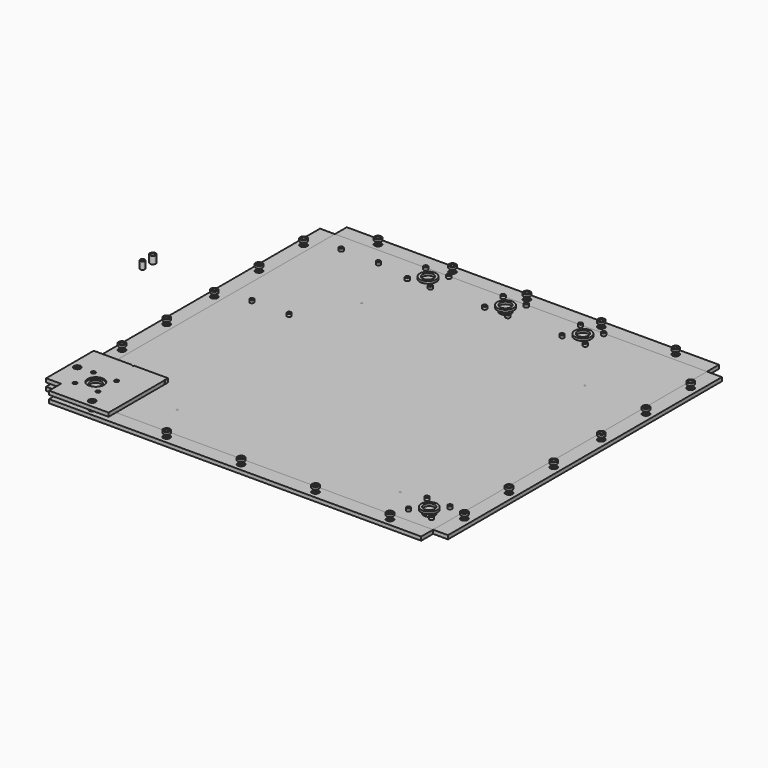
from build123d import *

# Parameters (mm, degrees)
F0_R      = 1.6
F0_R_2    = 2.6
F0_R_3    = 7.5
F0_R_4    = 1.25
F2_DEPTH  = 5
F3_R      = 2.75
F3_R_2    = 1.6
F3_R_3    = 4.6
F3_R_4    = 2.6
F4_DEPTH  = 1.5
F3_R_5    = 11
F3_R_6    = 7.5
F5_DEPTH  = 2
F6_R      = 3
F6_R_2    = 1.6
F7_DEPTH  = 5
F6_R_3    = 4
F6_R_4    = 2.6
F8_DEPTH  = 10
F10_W     = 500
F10_H     = 460
F10_R     = 7.5
F10_R_2   = 1.25
F10_W_2   = 65
F10_H_2   = 280
F11_DEPTH = 5
F12_DEPTH = 3
F14_R     = 4.6
F14_R_2   = 1.25
F14_R_3   = 2.75
F14_R_4   = 11
F15_DEPTH = 5


with BuildPart() as f2:
    # F0 (on Top) → F2 (new body)
    with BuildSketch(Plane.XY):
        Polygon((12.6355909109, 329.2870461196), (-237.3644090891, 329.2870461196), (-237.3644090891, 309.2870461196), (-257.3644090891, 309.2870461196), (-257.3644090891, -150.7129538804), (-237.3644090891, -150.7129538804), (-237.3644090891, -170.7129538804), (262.6355909109, -170.7129538804), (262.6355909109, -150.7129538804), (282.6355909109, -150.7129538804), (282.6355909109, 79.2870461196), (282.6355909109, 309.2870461196), (262.6355909109, 309.2870461196), (262.6355909109, 329.2870461196), align=None)
        with Locations((-226.8644090891, -140.2129538804)):
            Circle(F0_R, mode=Mode.SUBTRACT)
        with Locations((-195.8644090891, -140.2129538804)):
            Circle(F0_R, mode=Mode.SUBTRACT)
        with Locations((-247.3644090891, -110.7129538804)):
            Circle(F0_R_2, mode=Mode.SUBTRACT)
        with Locations((-226.8644090891, -109.2129538804)):
            Circle(F0_R, mode=Mode.SUBTRACT)
        with Locations((-211.3644090891, -124.7129538804)):
            Circle(F0_R_3, mode=Mode.SUBTRACT)
        with Locations((-195.8644090891, -109.2129538804)):
            Circle(F0_R, mode=Mode.SUBTRACT)
        with Locations((-187.3644090891, -160.7129538804)):
            Circle(F0_R_2, mode=Mode.SUBTRACT)
        with Locations((-204.3644090891, -70.8129538804)):
            Circle(F0_R_4, mode=Mode.SUBTRACT)
        with Locations((-156.6644090891, -77.1629538804)):
            Circle(F0_R_4, mode=Mode.SUBTRACT)
        with Locations((-87.3644090891, -160.7129538804)):
            Circle(F0_R_2, mode=Mode.SUBTRACT)
        with Locations((-247.3644090891, -35.7129538804)):
            Circle(F0_R_2, mode=Mode.SUBTRACT)
        with Locations((-204.3644090891, 4.1370461196)):
            Circle(F0_R_4, mode=Mode.SUBTRACT)
        with Locations((-156.6644090891, 5.3870461196)):
            Circle(F0_R_4, mode=Mode.SUBTRACT)
        with Locations((-247.3644090891, 39.2870461196)):
            Circle(F0_R_2, mode=Mode.SUBTRACT)
        with Locations((12.6355909109, -160.7129538804)):
            Circle(F0_R_2, mode=Mode.SUBTRACT)
        with Locations((112.6355909109, -160.7129538804)):
            Circle(F0_R_2, mode=Mode.SUBTRACT)
        with Locations((212.6355909109, -160.7129538804)):
            Circle(F0_R_2, mode=Mode.SUBTRACT)
        with Locations((221.1355909109, -140.2129538804)):
            Circle(F0_R, mode=Mode.SUBTRACT)
        with Locations((252.1355909109, -140.2129538804)):
            Circle(F0_R, mode=Mode.SUBTRACT)
        with Locations((236.6355909109, -124.7129538804)):
            Circle(F0_R_3, mode=Mode.SUBTRACT)
        with Locations((221.1355909109, -109.2129538804)):
            Circle(F0_R, mode=Mode.SUBTRACT)
        with Locations((252.1355909109, -109.2129538804)):
            Circle(F0_R, mode=Mode.SUBTRACT)
        with Locations((272.6355909109, -110.7129538804)):
            Circle(F0_R_2, mode=Mode.SUBTRACT)
        with Locations((272.6355909109, -35.7129538804)):
            Circle(F0_R_2, mode=Mode.SUBTRACT)
        with Locations((272.6355909109, 39.2870461196)):
            Circle(F0_R_2, mode=Mode.SUBTRACT)
        with Locations((-247.3644090891, 119.2870461196)):
            Circle(F0_R_2, mode=Mode.SUBTRACT)
        with Locations((-202.8644090891, 126.7870461196)):
            Circle(F0_R, mode=Mode.SUBTRACT)
        with Locations((-152.8644090891, 126.7870461196)):
            Circle(F0_R, mode=Mode.SUBTRACT)
        with Locations((-247.3644090891, 194.2870461196)):
            Circle(F0_R_2, mode=Mode.SUBTRACT)
        with Locations((-247.3644090891, 269.2870461196)):
            Circle(F0_R_2, mode=Mode.SUBTRACT)
        with Locations((-202.8644090891, 276.7870461196)):
            Circle(F0_R, mode=Mode.SUBTRACT)
        with Locations((-152.8644090891, 276.7870461196)):
            Circle(F0_R, mode=Mode.SUBTRACT)
        with Locations((-187.3644090891, 319.2870461196)):
            Circle(F0_R_2, mode=Mode.SUBTRACT)
        with Locations((-106.8644090891, 267.7870461196)):
            Circle(F0_R, mode=Mode.SUBTRACT)
        with Locations((-91.3644090891, 283.2870461196)):
            Circle(F0_R_3, mode=Mode.SUBTRACT)
        with Locations((-75.8644090891, 267.7870461196)):
            Circle(F0_R, mode=Mode.SUBTRACT)
        with Locations((-106.8644090891, 298.7870461196)):
            Circle(F0_R, mode=Mode.SUBTRACT)
        with Locations((-75.8644090891, 298.7870461196)):
            Circle(F0_R, mode=Mode.SUBTRACT)
        with Locations((-87.3644090891, 319.2870461196)):
            Circle(F0_R_2, mode=Mode.SUBTRACT)
        with Locations((-2.8644090891, 267.7870461196)):
            Circle(F0_R, mode=Mode.SUBTRACT)
        with Locations((-2.8644090891, 298.7870461196)):
            Circle(F0_R, mode=Mode.SUBTRACT)
        with Locations((272.6355909109, 119.2870461196)):
            Circle(F0_R_2, mode=Mode.SUBTRACT)
        with Locations((272.6355909109, 194.2870461196)):
            Circle(F0_R_2, mode=Mode.SUBTRACT)
        with Locations((28.1355909109, 267.7870461196)):
            Circle(F0_R, mode=Mode.SUBTRACT)
        with Locations((12.6355909109, 283.2870461196)):
            Circle(F0_R_3, mode=Mode.SUBTRACT)
        with Locations((28.1355909109, 298.7870461196)):
            Circle(F0_R, mode=Mode.SUBTRACT)
        with Locations((12.6355909109, 319.2870461196)):
            Circle(F0_R_2, mode=Mode.SUBTRACT)
        with Locations((101.1355909109, 267.7870461196)):
            Circle(F0_R, mode=Mode.SUBTRACT)
        with Locations((132.1355909109, 267.7870461196)):
            Circle(F0_R, mode=Mode.SUBTRACT)
        with Locations((116.6355909109, 283.2870461196)):
            Circle(F0_R_3, mode=Mode.SUBTRACT)
        with Locations((101.1355909109, 298.7870461196)):
            Circle(F0_R, mode=Mode.SUBTRACT)
        with Locations((112.6355909109, 319.2870461196)):
            Circle(F0_R_2, mode=Mode.SUBTRACT)
        with Locations((132.1355909109, 298.7870461196)):
            Circle(F0_R, mode=Mode.SUBTRACT)
        with Locations((212.6355909109, 319.2870461196)):
            Circle(F0_R_2, mode=Mode.SUBTRACT)
        with Locations((272.6355909109, 269.2870461196)):
            Circle(F0_R_2, mode=Mode.SUBTRACT)
    extrude(amount=F2_DEPTH)

    # F3 (on face) → F4 (cut)
    with BuildSketch(Plane.XY.offset(5)):
        with Locations((-202.8644090891, 276.7870461196)):
            Circle(F3_R)
        with Locations((-202.8644090891, 276.7870461196)):
            Circle(F3_R_2, mode=Mode.SUBTRACT)
        with Locations((-152.8644090891, 276.7870461196)):
            Circle(F3_R)
        with Locations((-152.8644090891, 276.7870461196)):
            Circle(F3_R_2, mode=Mode.SUBTRACT)
        with Locations((-106.8644090891, 267.7870461196)):
            Circle(F3_R)
        with Locations((-106.8644090891, 267.7870461196)):
            Circle(F3_R_2, mode=Mode.SUBTRACT)
        with Locations((272.6355909109, 269.2870461196)):
            Circle(F3_R_3)
        with Locations((272.6355909109, 269.2870461196)):
            Circle(F3_R_4, mode=Mode.SUBTRACT)
        with Locations((-106.8644090891, 298.7870461196)):
            Circle(F3_R)
        with Locations((-106.8644090891, 298.7870461196)):
            Circle(F3_R_2, mode=Mode.SUBTRACT)
        with Locations((-75.8644090891, 298.7870461196)):
            Circle(F3_R)
        with Locations((-75.8644090891, 298.7870461196)):
            Circle(F3_R_2, mode=Mode.SUBTRACT)
        with Locations((-75.8644090891, 267.7870461196)):
            Circle(F3_R)
        with Locations((-75.8644090891, 267.7870461196)):
            Circle(F3_R_2, mode=Mode.SUBTRACT)
        with Locations((101.1355909109, 298.7870461196)):
            Circle(F3_R)
        with Locations((101.1355909109, 298.7870461196)):
            Circle(F3_R_2, mode=Mode.SUBTRACT)
        with Locations((101.1355909109, 267.7870461196)):
            Circle(F3_R)
        with Locations((101.1355909109, 267.7870461196)):
            Circle(F3_R_2, mode=Mode.SUBTRACT)
        with Locations((132.1355909109, 298.7870461196)):
            Circle(F3_R)
        with Locations((132.1355909109, 298.7870461196)):
            Circle(F3_R_2, mode=Mode.SUBTRACT)
        with Locations((-202.8644090891, 126.7870461196)):
            Circle(F3_R)
        with Locations((-202.8644090891, 126.7870461196)):
            Circle(F3_R_2, mode=Mode.SUBTRACT)
        with Locations((-152.8644090891, 126.7870461196)):
            Circle(F3_R)
        with Locations((-152.8644090891, 126.7870461196)):
            Circle(F3_R_2, mode=Mode.SUBTRACT)
        with Locations((-187.3644090891, -160.7129538804)):
            Circle(F3_R_3)
        with Locations((-187.3644090891, -160.7129538804)):
            Circle(F3_R_4, mode=Mode.SUBTRACT)
        with Locations((-87.3644090891, -160.7129538804)):
            Circle(F3_R_3)
        with Locations((-87.3644090891, -160.7129538804)):
            Circle(F3_R_4, mode=Mode.SUBTRACT)
        with Locations((12.6355909109, -160.7129538804)):
            Circle(F3_R_3)
        with Locations((12.6355909109, -160.7129538804)):
            Circle(F3_R_4, mode=Mode.SUBTRACT)
        with Locations((112.6355909109, -160.7129538804)):
            Circle(F3_R_3)
        with Locations((112.6355909109, -160.7129538804)):
            Circle(F3_R_4, mode=Mode.SUBTRACT)
        with Locations((-195.8644090891, -109.2129538804)):
            Circle(F3_R)
        with Locations((-195.8644090891, -109.2129538804)):
            Circle(F3_R_2, mode=Mode.SUBTRACT)
        with Locations((-226.8644090891, -109.2129538804)):
            Circle(F3_R)
        with Locations((-226.8644090891, -109.2129538804)):
            Circle(F3_R_2, mode=Mode.SUBTRACT)
        with Locations((-226.8644090891, -140.2129538804)):
            Circle(F3_R)
        with Locations((-226.8644090891, -140.2129538804)):
            Circle(F3_R_2, mode=Mode.SUBTRACT)
        with Locations((-195.8644090891, -140.2129538804)):
            Circle(F3_R)
        with Locations((-195.8644090891, -140.2129538804)):
            Circle(F3_R_2, mode=Mode.SUBTRACT)
        with Locations((272.6355909109, 39.2870461196)):
            Circle(F3_R_3)
        with Locations((272.6355909109, 39.2870461196)):
            Circle(F3_R_4, mode=Mode.SUBTRACT)
        with Locations((272.6355909109, -35.7129538804)):
            Circle(F3_R_3)
        with Locations((272.6355909109, -35.7129538804)):
            Circle(F3_R_4, mode=Mode.SUBTRACT)
        with Locations((272.6355909109, -110.7129538804)):
            Circle(F3_R_3)
        with Locations((272.6355909109, -110.7129538804)):
            Circle(F3_R_4, mode=Mode.SUBTRACT)
        with Locations((221.1355909109, -109.2129538804)):
            Circle(F3_R)
        with Locations((221.1355909109, -109.2129538804)):
            Circle(F3_R_2, mode=Mode.SUBTRACT)
        with Locations((252.1355909109, -140.2129538804)):
            Circle(F3_R)
        with Locations((252.1355909109, -140.2129538804)):
            Circle(F3_R_2, mode=Mode.SUBTRACT)
        with Locations((221.1355909109, -140.2129538804)):
            Circle(F3_R)
        with Locations((221.1355909109, -140.2129538804)):
            Circle(F3_R_2, mode=Mode.SUBTRACT)
        with Locations((252.1355909109, -109.2129538804)):
            Circle(F3_R)
        with Locations((252.1355909109, -109.2129538804)):
            Circle(F3_R_2, mode=Mode.SUBTRACT)
        with Locations((272.6355909109, 119.2870461196)):
            Circle(F3_R_3)
        with Locations((272.6355909109, 119.2870461196)):
            Circle(F3_R_4, mode=Mode.SUBTRACT)
        with Locations((272.6355909109, 194.2870461196)):
            Circle(F3_R_3)
        with Locations((272.6355909109, 194.2870461196)):
            Circle(F3_R_4, mode=Mode.SUBTRACT)
        with Locations((132.1355909109, 267.7870461196)):
            Circle(F3_R)
        with Locations((132.1355909109, 267.7870461196)):
            Circle(F3_R_2, mode=Mode.SUBTRACT)
        with Locations((212.6355909109, -160.7129538804)):
            Circle(F3_R_3)
        with Locations((212.6355909109, -160.7129538804)):
            Circle(F3_R_4, mode=Mode.SUBTRACT)
        with Locations((-2.8644090891, 298.7870461196)):
            Circle(F3_R)
        with Locations((-2.8644090891, 298.7870461196)):
            Circle(F3_R_2, mode=Mode.SUBTRACT)
        with Locations((28.1355909109, 298.7870461196)):
            Circle(F3_R)
        with Locations((28.1355909109, 298.7870461196)):
            Circle(F3_R_2, mode=Mode.SUBTRACT)
        with Locations((28.1355909109, 267.7870461196)):
            Circle(F3_R)
        with Locations((28.1355909109, 267.7870461196)):
            Circle(F3_R_2, mode=Mode.SUBTRACT)
        with Locations((-2.8644090891, 267.7870461196)):
            Circle(F3_R)
        with Locations((-2.8644090891, 267.7870461196)):
            Circle(F3_R_2, mode=Mode.SUBTRACT)
    extrude(amount=-F4_DEPTH, mode=Mode.SUBTRACT)

    # F3 (on face) → F5 (cut)
    with BuildSketch(Plane.XY.offset(5)):
        with Locations((-211.3644090891, -124.7129538804)):
            Circle(F3_R_5)
        with Locations((-211.3644090891, -124.7129538804)):
            Circle(F3_R_6, mode=Mode.SUBTRACT)
        with Locations((236.6355909109, -124.7129538804)):
            Circle(F3_R_5)
        with Locations((236.6355909109, -124.7129538804)):
            Circle(F3_R_6, mode=Mode.SUBTRACT)
        with Locations((116.6355909109, 283.2870461196)):
            Circle(F3_R_5)
        with Locations((116.6355909109, 283.2870461196)):
            Circle(F3_R_6, mode=Mode.SUBTRACT)
        with Locations((-91.3644090891, 283.2870461196)):
            Circle(F3_R_5)
        with Locations((-91.3644090891, 283.2870461196)):
            Circle(F3_R_6, mode=Mode.SUBTRACT)
        with Locations((12.6355909109, 283.2870461196)):
            Circle(F3_R_5)
        with Locations((12.6355909109, 283.2870461196)):
            Circle(F3_R_6, mode=Mode.SUBTRACT)
        with Locations((-247.3644090891, 269.2870461196)):
            Circle(F3_R_3)
        with Locations((-247.3644090891, 269.2870461196)):
            Circle(F3_R_4, mode=Mode.SUBTRACT)
        with Locations((-187.3644090891, 319.2870461196)):
            Circle(F3_R_3)
        with Locations((-187.3644090891, 319.2870461196)):
            Circle(F3_R_4, mode=Mode.SUBTRACT)
        with Locations((-87.3644090891, 319.2870461196)):
            Circle(F3_R_3)
        with Locations((-87.3644090891, 319.2870461196)):
            Circle(F3_R_4, mode=Mode.SUBTRACT)
        with Locations((12.6355909109, 319.2870461196)):
            Circle(F3_R_3)
        with Locations((12.6355909109, 319.2870461196)):
            Circle(F3_R_4, mode=Mode.SUBTRACT)
        with Locations((112.6355909109, 319.2870461196)):
            Circle(F3_R_3)
        with Locations((112.6355909109, 319.2870461196)):
            Circle(F3_R_4, mode=Mode.SUBTRACT)
        with Locations((212.6355909109, 319.2870461196)):
            Circle(F3_R_3)
        with Locations((212.6355909109, 319.2870461196)):
            Circle(F3_R_4, mode=Mode.SUBTRACT)
        with Locations((272.6355909109, 269.2870461196)):
            Circle(F3_R_3)
        with Locations((272.6355909109, 269.2870461196)):
            Circle(F3_R_4, mode=Mode.SUBTRACT)
        with Locations((-247.3644090891, 194.2870461196)):
            Circle(F3_R_3)
        with Locations((-247.3644090891, 194.2870461196)):
            Circle(F3_R_4, mode=Mode.SUBTRACT)
        with Locations((-247.3644090891, 119.2870461196)):
            Circle(F3_R_3)
        with Locations((-247.3644090891, 119.2870461196)):
            Circle(F3_R_4, mode=Mode.SUBTRACT)
        with Locations((-247.3644090891, 39.2870461196)):
            Circle(F3_R_3)
        with Locations((-247.3644090891, 39.2870461196)):
            Circle(F3_R_4, mode=Mode.SUBTRACT)
        with Locations((-247.3644090891, -35.7129538804)):
            Circle(F3_R_3)
        with Locations((-247.3644090891, -35.7129538804)):
            Circle(F3_R_4, mode=Mode.SUBTRACT)
        with Locations((-247.3644090891, -110.7129538804)):
            Circle(F3_R_3)
        with Locations((-247.3644090891, -110.7129538804)):
            Circle(F3_R_4, mode=Mode.SUBTRACT)
        with Locations((-187.3644090891, -160.7129538804)):
            Circle(F3_R_3)
        with Locations((-187.3644090891, -160.7129538804)):
            Circle(F3_R_4, mode=Mode.SUBTRACT)
        with Locations((-87.3644090891, -160.7129538804)):
            Circle(F3_R_3)
        with Locations((-87.3644090891, -160.7129538804)):
            Circle(F3_R_4, mode=Mode.SUBTRACT)
        with Locations((12.6355909109, -160.7129538804)):
            Circle(F3_R_3)
        with Locations((12.6355909109, -160.7129538804)):
            Circle(F3_R_4, mode=Mode.SUBTRACT)
        with Locations((112.6355909109, -160.7129538804)):
            Circle(F3_R_3)
        with Locations((112.6355909109, -160.7129538804)):
            Circle(F3_R_4, mode=Mode.SUBTRACT)
        with Locations((272.6355909109, 39.2870461196)):
            Circle(F3_R_3)
        with Locations((272.6355909109, 39.2870461196)):
            Circle(F3_R_4, mode=Mode.SUBTRACT)
        with Locations((272.6355909109, -35.7129538804)):
            Circle(F3_R_3)
        with Locations((272.6355909109, -35.7129538804)):
            Circle(F3_R_4, mode=Mode.SUBTRACT)
        with Locations((272.6355909109, -110.7129538804)):
            Circle(F3_R_3)
        with Locations((272.6355909109, -110.7129538804)):
            Circle(F3_R_4, mode=Mode.SUBTRACT)
        with Locations((272.6355909109, 119.2870461196)):
            Circle(F3_R_3)
        with Locations((272.6355909109, 119.2870461196)):
            Circle(F3_R_4, mode=Mode.SUBTRACT)
        with Locations((272.6355909109, 194.2870461196)):
            Circle(F3_R_3)
        with Locations((272.6355909109, 194.2870461196)):
            Circle(F3_R_4, mode=Mode.SUBTRACT)
        with Locations((212.6355909109, -160.7129538804)):
            Circle(F3_R_3)
        with Locations((212.6355909109, -160.7129538804)):
            Circle(F3_R_4, mode=Mode.SUBTRACT)
        with Locations((272.6355909109, -110.7129538804)):
            Circle(F3_R_4)
        with Locations((212.6355909109, -160.7129538804)):
            Circle(F3_R_4)
        with Locations((272.6355909109, -35.7129538804)):
            Circle(F3_R_4)
        with Locations((112.6355909109, -160.7129538804)):
            Circle(F3_R_4)
        with Locations((272.6355909109, 39.2870461196)):
            Circle(F3_R_4)
        with Locations((272.6355909109, 119.2870461196)):
            Circle(F3_R_4)
        with Locations((272.6355909109, 194.2870461196)):
            Circle(F3_R_4)
        with Locations((272.6355909109, 269.2870461196)):
            Circle(F3_R_4)
        with Locations((-187.3644090891, -160.7129538804)):
            Circle(F3_R_4)
        with Locations((-87.3644090891, -160.7129538804)):
            Circle(F3_R_4)
        with Locations((12.6355909109, -160.7129538804)):
            Circle(F3_R_4)
    extrude(amount=-F5_DEPTH, mode=Mode.SUBTRACT)


with BuildPart() as f7:
    # F6 (on Top) → F7 (new body)
    with BuildSketch(Plane.XY):
        with Locations((-351.8798351288, 129.4269926766)):
            Circle(F6_R)
        with Locations((-351.8798351288, 129.4269926766)):
            Circle(F6_R_2, mode=Mode.SUBTRACT)
    extrude(amount=F7_DEPTH)


with BuildPart() as f7b:
    # F6 (on Top) → F7, piece 2 (new body)
    with BuildSketch(Plane.XY):
        with Locations((-351.8798351288, 146.7694063903)):
            Circle(F6_R_3)
        with Locations((-351.8798351288, 146.7694063903)):
            Circle(F6_R_4, mode=Mode.SUBTRACT)
    extrude(amount=F7_DEPTH)


with BuildPart() as f8:
    # F6 (on Top) → F8 (new body)
    with BuildSketch(Plane.XY):
        with Locations((-351.8798351288, 146.7694063903)):
            Circle(F6_R_3)
        with Locations((-351.8798351288, 146.7694063903)):
            Circle(F6_R_4, mode=Mode.SUBTRACT)
    extrude(amount=F8_DEPTH)


with BuildPart() as f8b:
    # F6 (on Top) → F8, piece 2 (new body)
    with BuildSketch(Plane.XY):
        with Locations((-351.8798351288, 129.4269926766)):
            Circle(F6_R)
        with Locations((-351.8798351288, 129.4269926766)):
            Circle(F6_R_2, mode=Mode.SUBTRACT)
    extrude(amount=F8_DEPTH)


with BuildPart() as f11:
    # F10 (on face) → F11 (new body)
    with BuildSketch(Plane.XY):
        with Locations((12.6355909109, 79.2870461196)):
            Rectangle(F10_W, F10_H)
        with Locations((-211.3644090891, -124.7129538804)):
            Circle(F10_R, mode=Mode.SUBTRACT)
        with Locations((236.6355909109, -124.7129538804)):
            Circle(F10_R, mode=Mode.SUBTRACT)
        Polygon((-128.5639107227, -110.7129538804), (-127.3644090891, 209.2870461196), (192.6355909109, 209.2870461196), (192.6355909109, -110.7129538804), (-117.3644090891, -110.7129538804), align=None, mode=Mode.SUBTRACT)
        with Locations((12.6355909109, 283.2870461196)):
            Circle(F10_R, mode=Mode.SUBTRACT)
        Polygon((192.6355909109, 209.2870461196), (-127.3644090891, 209.2870461196), (-128.5639107227, -110.7129538804), (-117.3644090891, -110.7129538804), (192.6355909109, -110.7129538804), align=None)
        with Locations((-117.3644090891, -105.7129538804)):
            Circle(F10_R_2, mode=Mode.SUBTRACT)
        with Locations((-74.8644090891, 49.2870461196)):
            Rectangle(F10_W_2, F10_H_2, mode=Mode.SUBTRACT)
        with Locations((182.6355909109, -105.7129538804)):
            Circle(F10_R_2, mode=Mode.SUBTRACT)
        with Locations((-117.3644090891, 204.2870461196)):
            Circle(F10_R_2, mode=Mode.SUBTRACT)
        with Locations((182.6355909109, 204.2870461196)):
            Circle(F10_R_2, mode=Mode.SUBTRACT)
        with Locations((-74.8644090891, 49.2870461196)):
            Rectangle(F10_W_2, F10_H_2)
    extrude(amount=F11_DEPTH)


with BuildPart() as f12:
    # F10 (on face) → F12 (new body)
    with BuildSketch(Plane.XY):
        Polygon((192.6355909109, 209.2870461196), (-127.3644090891, 209.2870461196), (-128.5639107227, -110.7129538804), (-117.3644090891, -110.7129538804), (192.6355909109, -110.7129538804), align=None)
        with Locations((-117.3644090891, -105.7129538804)):
            Circle(F10_R_2, mode=Mode.SUBTRACT)
        with Locations((-74.8644090891, 49.2870461196)):
            Rectangle(F10_W_2, F10_H_2, mode=Mode.SUBTRACT)
        with Locations((182.6355909109, -105.7129538804)):
            Circle(F10_R_2, mode=Mode.SUBTRACT)
        with Locations((-117.3644090891, 204.2870461196)):
            Circle(F10_R_2, mode=Mode.SUBTRACT)
        with Locations((182.6355909109, 204.2870461196)):
            Circle(F10_R_2, mode=Mode.SUBTRACT)
        with Locations((-74.8644090891, 49.2870461196)):
            Rectangle(F10_W_2, F10_H_2)
    extrude(amount=F12_DEPTH)


with BuildPart() as f13_1:
    # F13: copy of F2
    add(f2.part.moved(Location((0, 0, 10))))

    # F14 (on face) → F15 (cut)
    with BuildSketch(Plane.XY.offset(15)):
        with BuildLine():
            Line((-203.1184155097, -70.7129538804), (-157.3644090891, -70.7129538804))
            Line((-157.3644090891, -70.7129538804), (-157.3644090891, -76.1273381216))
            ThreePointArc((-157.3644090891, -76.1273381216), (-156.0781071191, -76.0589837721), (-155.4144090891, -77.1629538804))
            ThreePointArc((-155.4144090891, -77.1629538804), (-156.0781071191, -78.2669239887), (-157.3644090891, -78.1985696393))
            Line((-157.3644090891, -78.1985696393), (-157.3644090891, -150.7129538804))
            Line((-157.3644090891, -150.7129538804), (-157.3644090891, -170.7129538804))
            Line((-157.3644090891, -170.7129538804), (262.6355909109, -170.7129538804))
            Line((262.6355909109, -170.7129538804), (262.6355909109, -150.7129538804))
            Line((262.6355909109, -150.7129538804), (282.6355909109, -150.7129538804))
            Line((282.6355909109, -150.7129538804), (282.6355909109, 309.2870461196))
            Line((282.6355909109, 309.2870461196), (262.6355909109, 309.2870461196))
            Line((262.6355909109, 309.2870461196), (262.6355909109, 329.2870461196))
            Line((262.6355909109, 329.2870461196), (-237.3644090891, 329.2870461196))
            Line((-237.3644090891, 329.2870461196), (-237.3644090891, 309.2870461196))
            Line((-237.3644090891, 309.2870461196), (-257.3644090891, 309.2870461196))
            Line((-257.3644090891, 309.2870461196), (-257.3644090891, -70.7129538804))
            Line((-257.3644090891, -70.7129538804), (-237.3644090891, -70.7129538804))
            Line((-237.3644090891, -70.7129538804), (-205.6104026685, -70.7129538804))
            ThreePointArc((-205.6104026685, -70.7129538804), (-204.3644090891, -69.5629538804), (-203.1184155097, -70.7129538804))
        make_face()
        with Locations((-87.3644090891, -160.7129538804)):
            Circle(F14_R, mode=Mode.SUBTRACT)
        with Locations((-247.3644090891, -35.7129538804)):
            Circle(F14_R, mode=Mode.SUBTRACT)
        with Locations((-204.3644090891, 4.1370461196)):
            Circle(F14_R_2, mode=Mode.SUBTRACT)
        with BuildLine():
            ThreePointArc((-157.3644090891, 4.3514303607), (-157.9144090891, 5.3870461196), (-157.3644090891, 6.4226618784))
            ThreePointArc((-157.3644090891, 6.4226618784), (-156.0781071191, 6.4910162279), (-155.4144090891, 5.3870461196))
            ThreePointArc((-155.4144090891, 5.3870461196), (-156.0781071191, 4.2830760113), (-157.3644090891, 4.3514303607))
        make_face(mode=Mode.SUBTRACT)
        with Locations((-247.3644090891, 39.2870461196)):
            Circle(F14_R, mode=Mode.SUBTRACT)
        with Locations((12.6355909109, -160.7129538804)):
            Circle(F14_R, mode=Mode.SUBTRACT)
        with Locations((112.6355909109, -160.7129538804)):
            Circle(F14_R, mode=Mode.SUBTRACT)
        with Locations((212.6355909109, -160.7129538804)):
            Circle(F14_R, mode=Mode.SUBTRACT)
        with Locations((221.1355909109, -140.2129538804)):
            Circle(F14_R_3, mode=Mode.SUBTRACT)
        with Locations((252.1355909109, -140.2129538804)):
            Circle(F14_R_3, mode=Mode.SUBTRACT)
        with Locations((236.6355909109, -124.7129538804)):
            Circle(F14_R_4, mode=Mode.SUBTRACT)
        with Locations((221.1355909109, -109.2129538804)):
            Circle(F14_R_3, mode=Mode.SUBTRACT)
        with Locations((252.1355909109, -109.2129538804)):
            Circle(F14_R_3, mode=Mode.SUBTRACT)
        with Locations((272.6355909109, -110.7129538804)):
            Circle(F14_R, mode=Mode.SUBTRACT)
        with Locations((272.6355909109, -35.7129538804)):
            Circle(F14_R, mode=Mode.SUBTRACT)
        with Locations((272.6355909109, 39.2870461196)):
            Circle(F14_R, mode=Mode.SUBTRACT)
        with Locations((-247.3644090891, 119.2870461196)):
            Circle(F14_R, mode=Mode.SUBTRACT)
        with Locations((-202.8644090891, 126.7870461196)):
            Circle(F14_R_3, mode=Mode.SUBTRACT)
        with Locations((-152.8644090891, 126.7870461196)):
            Circle(F14_R_3, mode=Mode.SUBTRACT)
        with Locations((-247.3644090891, 194.2870461196)):
            Circle(F14_R, mode=Mode.SUBTRACT)
        with Locations((-247.3644090891, 269.2870461196)):
            Circle(F14_R, mode=Mode.SUBTRACT)
        with Locations((-202.8644090891, 276.7870461196)):
            Circle(F14_R_3, mode=Mode.SUBTRACT)
        with Locations((-152.8644090891, 276.7870461196)):
            Circle(F14_R_3, mode=Mode.SUBTRACT)
        with Locations((-187.3644090891, 319.2870461196)):
            Circle(F14_R, mode=Mode.SUBTRACT)
        with Locations((-106.8644090891, 267.7870461196)):
            Circle(F14_R_3, mode=Mode.SUBTRACT)
        with Locations((-91.3644090891, 283.2870461196)):
            Circle(F14_R_4, mode=Mode.SUBTRACT)
        with Locations((-75.8644090891, 267.7870461196)):
            Circle(F14_R_3, mode=Mode.SUBTRACT)
        with Locations((-106.8644090891, 298.7870461196)):
            Circle(F14_R_3, mode=Mode.SUBTRACT)
        with Locations((-75.8644090891, 298.7870461196)):
            Circle(F14_R_3, mode=Mode.SUBTRACT)
        with Locations((-87.3644090891, 319.2870461196)):
            Circle(F14_R, mode=Mode.SUBTRACT)
        with Locations((-2.8644090891, 267.7870461196)):
            Circle(F14_R_3, mode=Mode.SUBTRACT)
        with Locations((-2.8644090891, 298.7870461196)):
            Circle(F14_R_3, mode=Mode.SUBTRACT)
        with Locations((272.6355909109, 119.2870461196)):
            Circle(F14_R, mode=Mode.SUBTRACT)
        with Locations((272.6355909109, 194.2870461196)):
            Circle(F14_R, mode=Mode.SUBTRACT)
        with Locations((28.1355909109, 267.7870461196)):
            Circle(F14_R_3, mode=Mode.SUBTRACT)
        with Locations((12.6355909109, 283.2870461196)):
            Circle(F14_R_4, mode=Mode.SUBTRACT)
        with Locations((28.1355909109, 298.7870461196)):
            Circle(F14_R_3, mode=Mode.SUBTRACT)
        with Locations((12.6355909109, 319.2870461196)):
            Circle(F14_R, mode=Mode.SUBTRACT)
        with Locations((101.1355909109, 267.7870461196)):
            Circle(F14_R_3, mode=Mode.SUBTRACT)
        with Locations((132.1355909109, 267.7870461196)):
            Circle(F14_R_3, mode=Mode.SUBTRACT)
        with Locations((116.6355909109, 283.2870461196)):
            Circle(F14_R_4, mode=Mode.SUBTRACT)
        with Locations((101.1355909109, 298.7870461196)):
            Circle(F14_R_3, mode=Mode.SUBTRACT)
        with Locations((112.6355909109, 319.2870461196)):
            Circle(F14_R, mode=Mode.SUBTRACT)
        with Locations((132.1355909109, 298.7870461196)):
            Circle(F14_R_3, mode=Mode.SUBTRACT)
        with Locations((212.6355909109, 319.2870461196)):
            Circle(F14_R, mode=Mode.SUBTRACT)
        with Locations((272.6355909109, 269.2870461196)):
            Circle(F14_R, mode=Mode.SUBTRACT)
    extrude(amount=-F15_DEPTH, mode=Mode.SUBTRACT)


solid = Compound([f2.part, f7.part, f7b.part, f8.part, f8b.part, f11.part, f12.part, f13_1.part])
